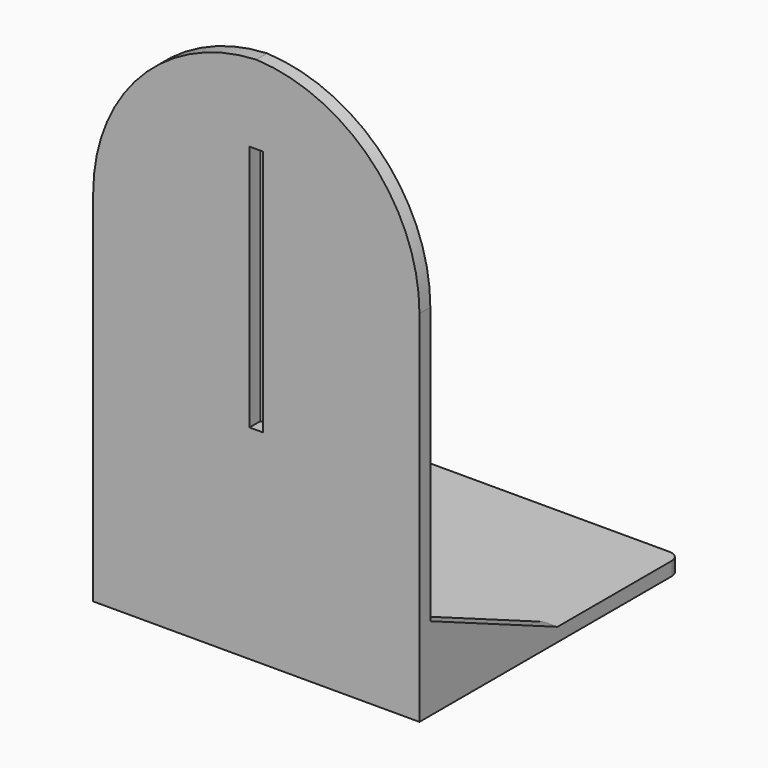
from build123d import *

# Parameters (mm, degrees)
F0_W        = 152.4
F0_H        = 152.4
F1_DEPTH    = 6.35
F2_W        = 152.4
F2_H        = 6.35
F3_DEPTH    = 241.3
F5_T1_DEPTH = 404.9366591478
F6_W        = 6.35
F6_H        = 115.4995709658
F7_DEPTH    = 25.4
F8_R        = 5.08
F9_DEPTH    = 6.35
F11_DEPTH   = 6.35


# Not quite as in the source:
# - a fillet or chamfer that OpenCascade refuses, or shapes differently, is made with other operations: its cross-section is extruded or revolved along the edge and cut away or added


with BuildPart() as f1:
    # F0 (on Top) → F1 (new body)
    with BuildSketch(Plane.XY):
        with Locations((2.7477228088, -4.3853670359)):
            Rectangle(F0_W, F0_H)
    extrude(amount=F1_DEPTH)

    # F2 (on face) → F3 (join)
    with BuildSketch(Plane.XY.offset(6.35)):
        with Locations((2.7477228088, -77.4103670359)):
            Rectangle(F2_W, F2_H)
    extrude(amount=F3_DEPTH)

    # F5: fillet of radius 79.7173318296 on 2 edges, made by hand

    # F5_s2 → F5_t1 (cut)
    with BuildSketch(Plane.XZ.offset(-125.057962538)):
        with BuildLine():
            ThreePointArc((-73.4522771912, 167.9326681704), (-50.1036112765, 224.3013340852), (6.2650546383, 247.65))
            Line((6.2650546383, 247.65), (-73.4522771912, 247.65))
            Line((-73.4522771912, 247.65), (-73.4522771912, 167.9326681704))
        make_face()
        with BuildLine():
            ThreePointArc((78.9477228088, 167.9326681704), (55.599056894, 224.3013340852), (-0.7696090208, 247.65))
            Line((-0.7696090208, 247.65), (78.9477228088, 247.65))
            Line((78.9477228088, 247.65), (78.9477228088, 167.9326681704))
        make_face()
    extrude(amount=F5_T1_DEPTH, mode=Mode.SUBTRACT)

    # F6 (on face) → F7 (cut)
    with BuildSketch(Plane.XZ.offset(80.5853670359)):
        with Locations((2.7477228088, 153.0246064067)):
            Rectangle(F6_W, F6_H)
    extrude(amount=-F7_DEPTH, mode=Mode.SUBTRACT)

    # F8
    f8_edges = [f1.edges().sort_by_distance(p)[0] for p in [
        (78.947723, 71.814633, 3.175),
        (-73.452277, 71.814633, 3.175),
    ]]
    fillet(f8_edges, radius=F8_R)

    # F4 (on face) → F9 (join)
    with BuildSketch(Plane.YZ.offset(78.9477228088)):
        Polygon((-74.2353670359, 6.35), (0, 6.35), (-74.2353670359, 38.8328842819), align=None)
    extrude(amount=-F9_DEPTH)

    # F10 (on face) → F11 (join)
    with BuildSketch(Plane(origin=(-73.4522771912, 0, 0), x_dir=(0, -1, 0), z_dir=(-1, 0, 0))):
        Polygon((74.2353670359, 6.35), (74.2353670359, 38.6480651796), (0, 6.35), align=None)
    extrude(amount=-F11_DEPTH)


solid = f1.part
